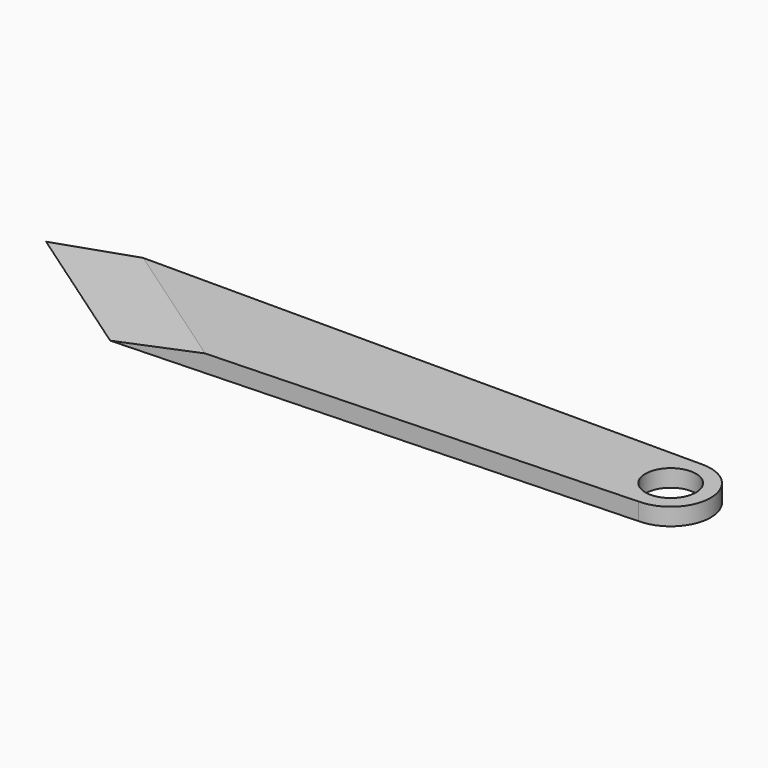
from build123d import *

# Parameters (mm, degrees)
F0_R     = 4.6477092711
F1_DEPTH = 3.175
F2_SIZE2 = 10.15999
F2_SIZE  = 3.17499


# Not quite as in the source:
# - a fillet or chamfer is up to 0.001 mm smaller than in the source, because OpenCascade refuses the exact size


with BuildPart() as f1:
    # F0 (on Top) → F1 (new body)
    with BuildSketch(Plane.XY):
        with BuildLine():
            Line((54.7894574702, 39.7151075304), (-65.8053308725, 39.7151075304))
            Line((-65.8053308725, 39.7151075304), (-39.4252166152, 21.4519556612))
            Line((-39.4252166152, 21.4519556612), (54.7894574702, 25.0102191872))
            ThreePointArc((54.7894574702, 25.0102191872), (62.1419016418, 32.3626633588), (54.7894574702, 39.7151075304))
        make_face()
        with Locations((54.7894574702, 32.3626633588)):
            Circle(F0_R, mode=Mode.SUBTRACT)
    extrude(amount=F1_DEPTH)

    # F2 (size 3.175 and 10.16 in the source; OpenCascade refuses exactly that, so slightly less here)
    f2_edges = [f1.edges().sort_by_distance(p)[0] for p in [
        (-52.615274, 30.583532, 3.175),
    ]]
    f2_side = f1.faces().sort_by_distance((-52.615274, 30.583532, 1.5875))[0]
    chamfer(f2_edges, length=F2_SIZE, length2=F2_SIZE2, reference=f2_side)


solid = f1.part
